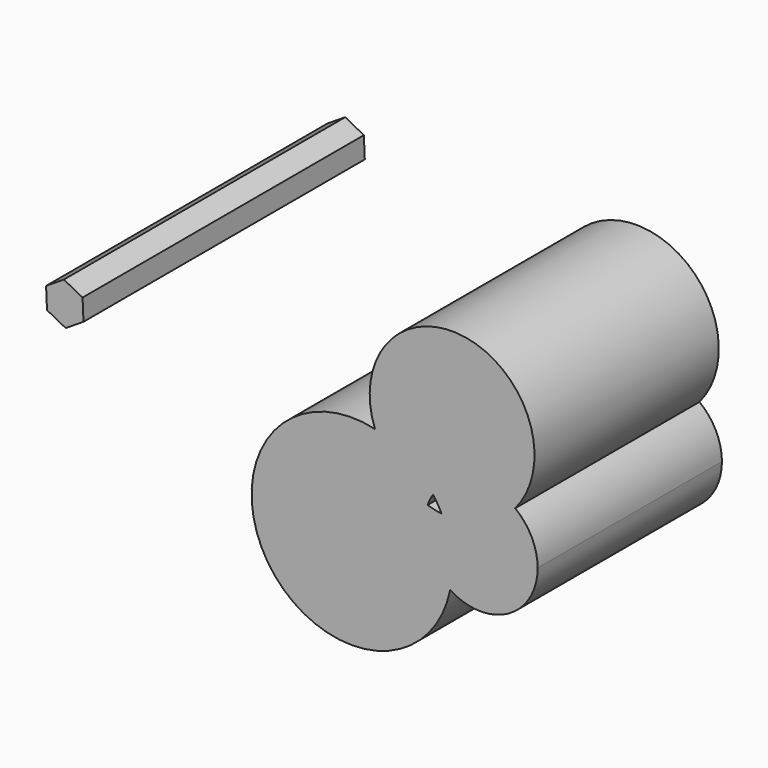
from build123d import *

# Parameters (mm, degrees)
F1_DEPTH = 114.808
F3_DEPTH = 175.26


with BuildPart() as f1:
    # F0 (on Front) → F1 (new body)
    with BuildSketch(Plane.XZ):
        with BuildLine():
            ThreePointArc((25.6628487822, -7.4808111298), (32.8172024659, 4.885626696), (35.3022317211, 18.9546775073))
            ThreePointArc((35.3022317211, 18.9546775073), (-13.0768212072, 59.3674402536), (-44.2324815618, 4.567358293))
            ThreePointArc((-44.2324815618, 4.567358293), (-28.0105833553, -2.4918355408), (-15.2659029767, -14.7619341979))
            ThreePointArc((-15.2659029767, -14.7619341979), (3.6055698097, -2.1673233144), (25.6628487822, -7.4808111298))
        make_face()
        with BuildLine():
            ThreePointArc((-15.2659029767, -14.7619341979), (-28.0105833553, -2.4918355408), (-44.2324815618, 4.567358293))
            ThreePointArc((-44.2324815618, 4.567358293), (-33.9881943736, -10.8809466008), (-17.9946564633, -20.2512341736))
            ThreePointArc((-17.9946564633, -20.2512341736), (-16.7793493314, -17.4324810717), (-15.2659029767, -14.7619341979))
        make_face()
        with BuildLine():
            ThreePointArc((-17.9946564633, -20.2512341736), (-33.9881943736, -10.8809466008), (-44.2324815618, 4.567358293))
            ThreePointArc((-44.2324815618, 4.567358293), (-97.7867193033, -71.0372404865), (-6.7479680143, -53.8309189616))
            ThreePointArc((-6.7479680143, -53.8309189616), (-18.2726677918, -39.0175902767), (-17.9946564633, -20.2512341736))
        make_face()
        with BuildLine():
            ThreePointArc((36.8622799555, -30.0298947841), (33.9082472391, -17.4413242511), (25.6628487822, -7.4808111298))
            ThreePointArc((25.6628487822, -7.4808111298), (9.1457659897, -19.3109785443), (-11.0207481957, -21.7764583426))
            ThreePointArc((-11.0207481957, -21.7764583426), (-7.1086795164, -32.609081399), (-5.781140064, -44.0496951342))
            ThreePointArc((-5.781140064, -44.0496951342), (-6.0234345779, -48.9641405721), (-6.7479680143, -53.8309189616))
            ThreePointArc((-6.7479680143, -53.8309189616), (22.1197578366, -54.8711028862), (36.8622799555, -30.0298947841))
        make_face()
        with BuildLine():
            ThreePointArc((-11.0207481957, -21.7764583426), (9.1457659897, -19.3109785443), (25.6628487822, -7.4808111298))
            ThreePointArc((25.6628487822, -7.4808111298), (3.6055698097, -2.1673233144), (-15.2659029767, -14.7619341979))
            ThreePointArc((-15.2659029767, -14.7619341979), (-12.9991883072, -18.181965113), (-11.0207481957, -21.7764583426))
        make_face()
        with BuildLine():
            ThreePointArc((-11.0207481957, -21.7764583426), (-14.5409053643, -21.165663233), (-17.9946564633, -20.2512341736))
            ThreePointArc((-17.9946564633, -20.2512341736), (-18.2726677918, -39.0175902767), (-6.7479680143, -53.8309189616))
            ThreePointArc((-6.7479680143, -53.8309189616), (-6.0234345779, -48.9641405721), (-5.781140064, -44.0496951342))
            ThreePointArc((-5.781140064, -44.0496951342), (-7.1086795164, -32.609081399), (-11.0207481957, -21.7764583426))
        make_face()
    extrude(amount=F1_DEPTH)


with BuildPart() as f3:
    # F2 (on Front) → F3 (new body)
    with BuildSketch(Plane.XZ):
        Polygon((-149.9888761281, 39.031247435), (-141.1276297332, 44.6808758994), (-141.5897283079, 55.1797546189), (-150.9130732776, 60.0290048739), (-159.7743196725, 54.3793764094), (-159.3122210978, 43.8804976899), align=None)
    extrude(amount=F3_DEPTH)


solid = Compound([f1.part, f3.part])
